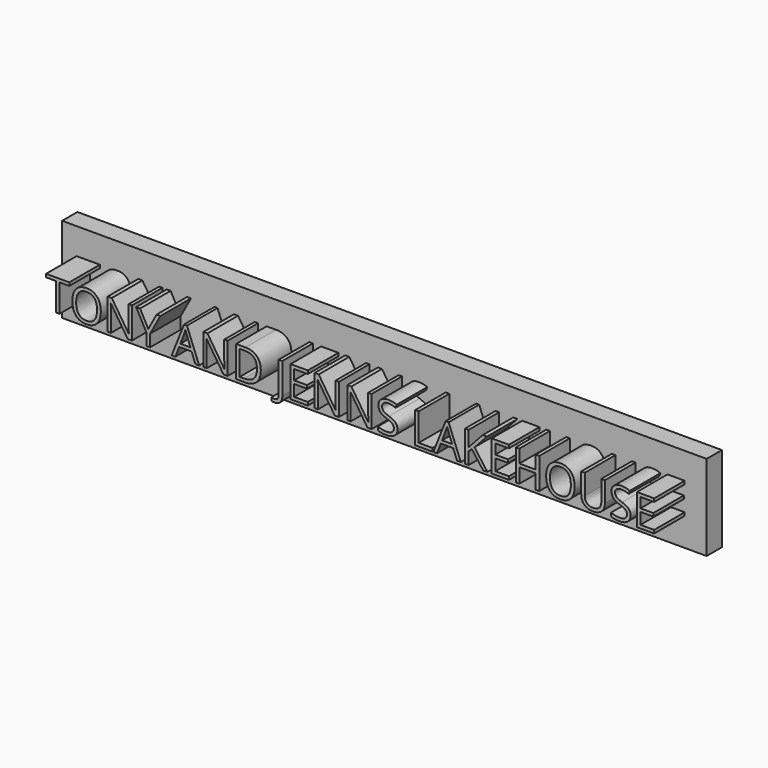
from build123d import *

# Parameters (mm, degrees)
F0_TEXT_SIZE = 14.4142226951
F1_DEPTH     = 12.7
F2_W         = 214.2447978258
F2_H         = 28.4395748749
F3_DEPTH     = 6.35


# Not quite as in the source:
# - Text() gives the source's letters only with a copy of the font that has no kerning and outlines rounded to 1/6400 em; it was checked with that copy


with BuildPart() as f1:
    # F0 (on Front) → F1 (new body)
    with BuildSketch(Plane.XZ):
        with Locations((-103.211565199, -4.9366150164)):
            Text('TONY AND JENNS LAKEHOUSE', F0_TEXT_SIZE, font='Open Sans', text_align=(TextAlign.LEFT, TextAlign.BOTTOM))
    extrude(amount=F1_DEPTH)


with BuildPart() as f3:
    # F2 (on Front) → F3 (new body)
    with BuildSketch(Plane.XZ):
        with Locations((-0.7834583521, -0.0947988592)):
            Rectangle(F2_W, F2_H)
    extrude(amount=-F3_DEPTH)


solid = Compound([f1.part, f3.part])
